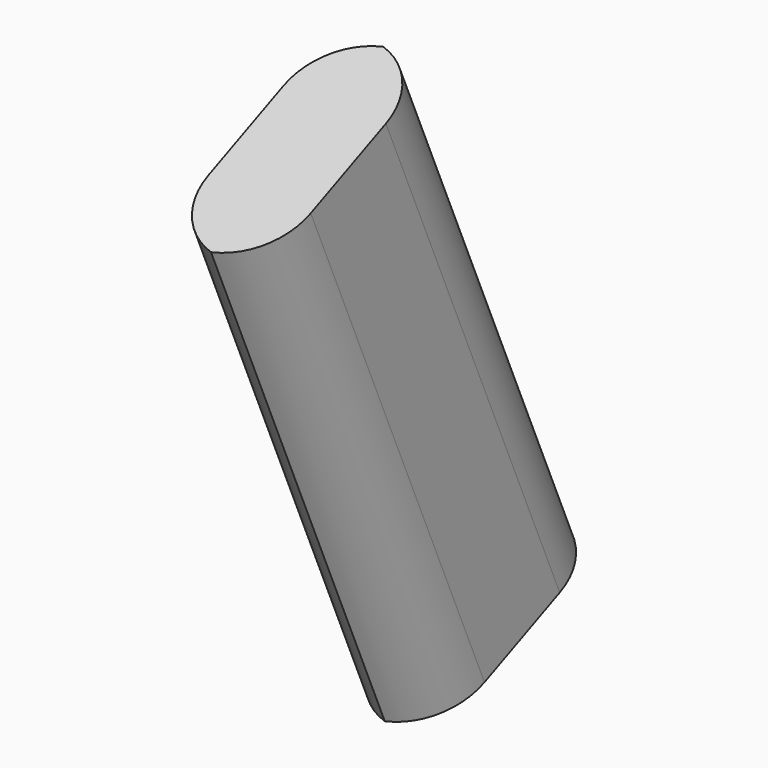
from build123d import *

# Parameters (mm, degrees)
F1_DEPTH    = 19.05
F2_T1_DEPTH = 165.1
F2_T3_DEPTH = 165.1


# Not quite as in the source:
# - a fillet or chamfer that OpenCascade refuses, or shapes differently, is made with other operations: its cross-section is extruded or revolved along the edge and cut away or added
# - a feature names something its author has since deleted; it is built from what else it names


with BuildPart() as f1:
    # F0 (on Right) → F1 (new body)
    with BuildSketch(Plane.YZ):
        Polygon((-36.6194384832, 94.9639305791), (3.7774763688, 1.7402786959), (44.5628240677, 19.4139289437), (4.1659092157, 112.6375808269), align=None)
    extrude(amount=F1_DEPTH)

    # F2: fillet of radius 12.7 on 4 edges, made by hand

    # F2_s2 → F2_t1 (cut)
    with BuildSketch(Plane(origin=(0, 12.5863228888, -29.0453612057), x_dir=(1, 0, 0), z_dir=(0, -0.3976074296, 0.9175556288))):
        with BuildLine():
            ThreePointArc((12.7, 48.6079924439), (3.7197438789, 44.888248565), (0, 35.9079924439))
            Line((0, 35.9079924439), (0, 48.6079924439))
            Line((0, 48.6079924439), (12.7, 48.6079924439))
        make_face()
        with BuildLine():
            ThreePointArc((6.35, 48.6079924439), (15.3302561211, 44.888248565), (19.05, 35.9079924439))
            Line((19.05, 35.9079924439), (19.05, 48.6079924439))
            Line((19.05, 48.6079924439), (6.35, 48.6079924439))
        make_face()
    extrude(amount=F2_T1_DEPTH, mode=Mode.SUBTRACT)

    # F2_s4 → F2_t3 (cut)
    with BuildSketch(Plane(origin=(0, -53.0586637457, 122.4430731045), x_dir=(1, 0, 0), z_dir=(0, 0.3976074296, -0.9175556288))):
        with BuildLine():
            ThreePointArc((12.7, -4.1579924439), (3.7197438789, -7.8777363228), (0, -16.8579924439))
            Line((0, -16.8579924439), (0, -4.1579924439))
            Line((0, -4.1579924439), (12.7, -4.1579924439))
        make_face()
        with BuildLine():
            ThreePointArc((6.35, -4.1579924439), (15.3302561211, -7.8777363228), (19.05, -16.8579924439))
            Line((19.05, -16.8579924439), (19.05, -4.1579924439))
            Line((19.05, -4.1579924439), (6.35, -4.1579924439))
        make_face()
    extrude(amount=F2_T3_DEPTH, mode=Mode.SUBTRACT)


solid = f1.part
